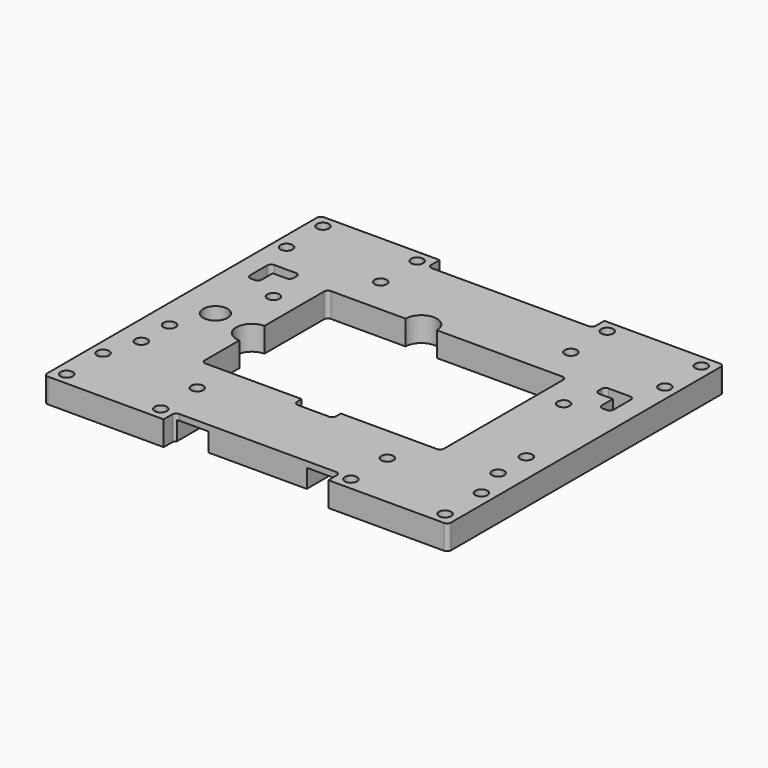
from build123d import *

# Parameters (mm, degrees)
F0_W      = 61
F0_H      = 40
F1_DEPTH  = 6.25
F2_R      = 1.55
F2_R_2    = 3.125
F3_DEPTH  = 25
F4_R      = 4
F4_W      = 10
F4_H      = 2.5
F5_DEPTH  = 25
F6_R      = 1
F8_DEPTH  = 4.75
F10_DEPTH = 1.75
F11_W     = 8
F11_H     = 11.5
F12_DEPTH = 1
F13_W     = 8
F13_H     = 8
F14_DEPTH = 1
F15_W     = 8
F15_H     = 4.5
F16_DEPTH = 1
F17_R     = 0.99999


# Not quite as in the source:
# - a fillet or chamfer is up to 0.001 mm smaller than in the source, because OpenCascade refuses the exact size


with BuildPart() as f1:
    # F0 (on Top) → F1 (new body)
    with BuildSketch(Plane.XY):
        Polygon((51.5, -44), (51.5, 44), (21, 44), (21, 40.25), (-21, 40.25), (-21, 44), (-51.5, 44), (-51.5, -44), (-21, -44), (-21, -40.25), (21, -40.25), (21, -44), align=None)
        Rectangle(F0_W, F0_H, mode=Mode.SUBTRACT)
    extrude(amount=F1_DEPTH)

    # F2 (on face) → F3 (cut)
    with BuildSketch(Plane.XY.offset(6.25)):
        with Locations((-48.25, 40.85)):
            Circle(F2_R)
        with Locations((-24.25, 40.85)):
            Circle(F2_R)
        with Locations((-24.25, 29.25)):
            Circle(F2_R)
        with Locations((-48.25, 29.25)):
            Circle(F2_R)
        with Locations((24.25, 40.85)):
            Circle(F2_R)
        with Locations((48.25, 40.85)):
            Circle(F2_R)
        with Locations((48.25, 29.25)):
            Circle(F2_R)
        with Locations((24.25, 29.25)):
            Circle(F2_R)
        with Locations((24.25, -29.25)):
            Circle(F2_R)
        with Locations((24.25, -40.85)):
            Circle(F2_R)
        with Locations((48.25, -29.25)):
            Circle(F2_R)
        with Locations((48.25, -40.85)):
            Circle(F2_R)
        with Locations((-24.25, -29.25)):
            Circle(F2_R)
        with Locations((-48.25, -29.25)):
            Circle(F2_R)
        with Locations((-48.25, -40.85)):
            Circle(F2_R)
        with Locations((-24.25, -40.85)):
            Circle(F2_R)
        Polygon((-38.875, 21.75), (-46.375, 21.75), (-46.375, 14.25), (-43.375, 14.25), (-43.375, 18.75), (-38.875, 18.75), align=None)
        Polygon((46.375, 21.75), (38.875, 21.75), (38.875, 18.75), (43.375, 18.75), (43.375, 14.25), (46.375, 14.25), align=None)
        with Locations((-37, 11)):
            Circle(F2_R)
        with Locations((37, 11)):
            Circle(F2_R)
        with Locations((-45.5, -11.5)):
            Circle(F2_R)
        with Locations((-45.5, -20.5)):
            Circle(F2_R)
        with Locations((45.5, -11.5)):
            Circle(F2_R)
        with Locations((45.5, -20.5)):
            Circle(F2_R)
        with Locations((-41.5, -1.875)):
            Circle(F2_R_2)
    extrude(amount=-F3_DEPTH, mode=Mode.SUBTRACT)

    # F4 (on face) → F5 (cut)
    with BuildSketch(Plane.XY.offset(6.25)):
        with Locations((-6.5, 20)):
            Circle(F4_R)
        with Locations((-30.5, -4)):
            Circle(F4_R)
        with Locations((0, -21.25)):
            Rectangle(F4_W, F4_H)
    extrude(amount=-F5_DEPTH, mode=Mode.SUBTRACT)

    # F6
    f6_edges = [f1.edges().sort_by_distance(p)[0] for p in [
        (51.5, 44, 3.125),
        (-21, 40.25, 3.125),
        (21, 40.25, 3.125),
        (-51.5, 44, 3.125),
        (46.375, 14.25, 3.125),
        (43.375, 14.25, 3.125),
        (38.875, 18.75, 3.125),
        (38.875, 21.75, 3.125),
        (46.375, 21.75, 3.125),
        (30.5, 20, 3.125),
        (-30.5, 20, 3.125),
        (-46.375, 21.75, 3.125),
        (-38.875, 21.75, 3.125),
        (-38.875, 18.75, 3.125),
        (-43.375, 14.25, 3.125),
        (-46.375, 14.25, 3.125),
        (-51.5, -44, 3.125),
        (21, -40.25, 3.125),
        (51.5, -44, 3.125),
        (-21, -40.25, 3.125),
        (-30.5, -20, 3.125),
        (-5, -22.5, 3.125),
        (30.5, -20, 3.125),
        (5, -22.5, 3.125),
    ]]
    fillet(f6_edges, radius=F6_R)

    # F7 (on face) → F8 (cut)
    with BuildSketch(Plane(origin=(0, 0, 0), x_dir=(1, 0, 0), z_dir=(0, 0, -1))):
        Polygon((27.75, -28.55), (27.75, -41.55), (30.25, -41.55), (30.25, -40.55), (42.25, -40.55), (42.25, -41.55), (44.75, -41.55), (44.75, -28.55), (42.25, -28.55), (42.25, -29.55), (30.25, -29.55), (30.25, -28.55), align=None)
        Polygon((30.25, 29.45), (42.25, 29.45), (42.25, 28.45), (44.75, 28.45), (44.75, 41.45), (42.25, 41.45), (42.25, 40.45), (30.25, 40.45), (30.25, 41.45), (27.75, 41.45), (27.75, 28.45), (30.25, 28.45), align=None)
        Polygon((-42.25, -40.55), (-30.25, -40.55), (-30.25, -41.55), (-27.75, -41.55), (-27.75, -28.55), (-30.25, -28.55), (-30.25, -29.55), (-42.25, -29.55), (-42.25, -28.55), (-44.75, -28.55), (-44.75, -41.55), (-42.25, -41.55), align=None)
        Polygon((-42.25, 29.45), (-30.25, 29.45), (-30.25, 28.45), (-27.75, 28.45), (-27.75, 41.45), (-30.25, 41.45), (-30.25, 40.45), (-42.25, 40.45), (-42.25, 41.45), (-44.75, 41.45), (-44.75, 28.45), (-42.25, 28.45), align=None)
    extrude(amount=-F8_DEPTH, mode=Mode.SUBTRACT)

    # F9 (on face) → F10 (cut)
    with BuildSketch(Plane(origin=(0, 0, 0), x_dir=(1, 0, 0), z_dir=(0, 0, -1))):
        Polygon((20.5, -40.25), (20.5, -26.25), (12.5, -26.25), (12.5, -40.25), (20.5, -41.25), align=None)
        Polygon((-12.5, -40.25), (-12.5, -26.25), (-20.5, -26.25), (-20.5, -40.25), (-20.5, -41.25), align=None)
        Polygon((12.5, 26.25), (20.5, 26.25), (20.5, 40.25), (20.5, 41.25), (12.5, 40.25), align=None)
        Polygon((-20.5, 26.25), (-12.5, 26.25), (-12.5, 40.25), (-20.5, 41.25), (-20.5, 40.25), align=None)
    extrude(amount=-F10_DEPTH, mode=Mode.SUBTRACT)

    # F11 (on face) → F12 (cut)
    with BuildSketch(Plane(origin=(0, 0, 1.75), x_dir=(1, 0, 0), z_dir=(0, 0, -1))):
        with Locations((16.5, -35.5)):
            Rectangle(F11_W, F11_H)
        with Locations((-16.5, -35.5)):
            Rectangle(F11_W, F11_H)
        with Locations((16.5, 35.5)):
            Rectangle(F11_W, F11_H)
        with Locations((-16.5, 35.5)):
            Rectangle(F11_W, F11_H)
    extrude(amount=-F12_DEPTH, mode=Mode.SUBTRACT)

    # F13 (on face) → F14 (cut)
    with BuildSketch(Plane(origin=(0, 0, 2.75), x_dir=(1, 0, 0), z_dir=(0, 0, -1))):
        with Locations((16.5, -37.25)):
            Rectangle(F13_W, F13_H)
        with Locations((-16.5, -37.25)):
            Rectangle(F13_W, F13_H)
        with Locations((16.5, 37.25)):
            Rectangle(F13_W, F13_H)
        with Locations((-16.5, 37.25)):
            Rectangle(F13_W, F13_H)
    extrude(amount=-F14_DEPTH, mode=Mode.SUBTRACT)

    # F15 (on face) → F16 (cut)
    with BuildSketch(Plane(origin=(0, 0, 3.75), x_dir=(1, 0, 0), z_dir=(0, 0, -1))):
        with Locations((16.5, -39)):
            Rectangle(F15_W, F15_H)
        with Locations((-16.5, -39)):
            Rectangle(F15_W, F15_H)
        with Locations((16.5, 39)):
            Rectangle(F15_W, F15_H)
        with Locations((-16.5, 39)):
            Rectangle(F15_W, F15_H)
    extrude(amount=-F16_DEPTH, mode=Mode.SUBTRACT)

    # F17 (radius 1 in the source; OpenCascade refuses exactly that, so slightly less here)
    f17_edges = [f1.edges().sort_by_distance(p)[0] for p in [
        (44.75, 41.55, 2.375),
        (30.25, 41.55, 2.375),
        (27.75, 41.55, 2.375),
        (42.25, 41.55, 2.375),
        (30.25, 28.55, 2.375),
        (44.75, 28.55, 2.375),
        (42.25, 28.55, 2.375),
        (27.75, 28.55, 2.375),
        (-44.75, 28.55, 2.375),
        (-30.25, 28.55, 2.375),
        (-42.25, 28.55, 2.375),
        (-27.75, 28.55, 2.375),
        (-30.25, 41.55, 2.375),
        (-44.75, 41.55, 2.375),
        (-27.75, 41.55, 2.375),
        (-42.25, 41.55, 2.375),
        (-27.75, -28.45, 2.375),
        (-42.25, -28.45, 2.375),
        (-30.25, -28.45, 2.375),
        (-44.75, -28.45, 2.375),
        (-44.75, -41.45, 2.375),
        (-30.25, -41.45, 2.375),
        (-42.25, -41.45, 2.375),
        (-27.75, -41.45, 2.375),
        (30.25, -41.45, 2.375),
        (44.75, -41.45, 2.375),
        (27.75, -41.45, 2.375),
        (42.25, -41.45, 2.375),
        (42.25, -28.45, 2.375),
        (27.75, -28.45, 2.375),
        (30.25, -28.45, 2.375),
        (44.75, -28.45, 2.375),
    ]]
    fillet(f17_edges, radius=F17_R)


solid = f1.part
